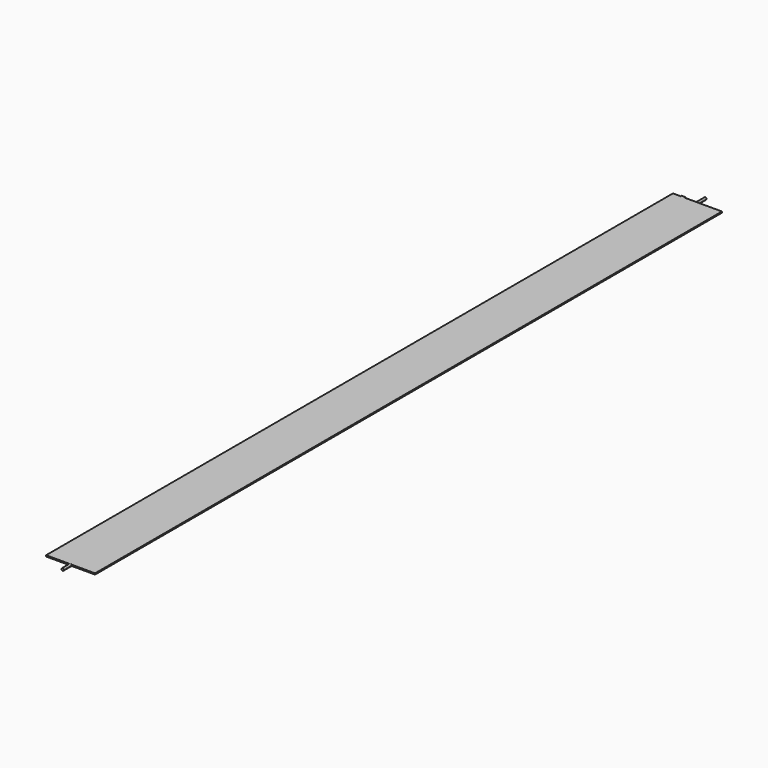
from build123d import *

# Parameters (mm, degrees)
F1_DEPTH = 3
F2_W     = 10
F2_H     = 3
F2_H_2   = 40
F2_R     = 1.5
F3_DEPTH = 3
F5_DEPTH = 25
F7_DEPTH = 25


# Not quite as in the source:
# - a feature names something its author has since deleted; it is built from what else it names


with BuildPart() as f1:
    # F0 (on Top) → F1 (new body)
    with BuildSketch(Plane.XY):
        Polygon((25.6095033884, 1855.804875493), (-34.3904966116, 1855.804875493), (-34.3904966116, -144.195124507), (25.6095033884, -144.195124507), (25.6095033884, -164.195124507), (30.6095033884, -164.195124507), (30.6095033884, -144.195124507), (90.6095033884, -144.195124507), (90.6095033884, 1855.804875493), (30.6095033884, 1855.804875493), (30.6095033884, 1875.804875493), (25.6095033884, 1875.804875493), align=None)
    extrude(amount=F1_DEPTH)

    # F2 (on face) → F3 (join)
    with BuildSketch(Plane(origin=(0, 1855.804875493, 0), x_dir=(-1, 0, 0), z_dir=(0, 1, 0))):
        with Locations((9.3904966116, 1.5)):
            Rectangle(F2_W, F2_H)
        with Locations((9.3904966116, -20)):
            Rectangle(F2_W, F2_H_2)
        with Locations((9.3904966116, -35)):
            Circle(F2_R, mode=Mode.SUBTRACT)
    extrude(amount=F3_DEPTH)

    # F4 (on face) → F5 (join)
    with BuildSketch(Plane.XZ.offset(144.195124507)):
        with BuildLine():
            Line((30.6095033884, 3), (30.7075795998, 3))
            ThreePointArc((30.7075795998, 3), (25.1095033884, 1.5), (30.7075795998, 0))
            Line((30.7075795998, 0), (30.6095033884, 0))
            Line((30.6095033884, 0), (30.6095033884, 3))
        make_face()
        with BuildLine():
            ThreePointArc((30.7075795998, 0), (31.0072808673, 0.7235428647), (31.1095033884, 1.5))
            ThreePointArc((31.1095033884, 1.5), (31.0072808673, 2.2764571353), (30.7075795998, 3))
            Line((30.7075795998, 3), (30.6095033884, 3))
            Line((30.6095033884, 3), (30.6095033884, 0))
            Line((30.6095033884, 0), (30.7075795998, 0))
        make_face()
    extrude(amount=F5_DEPTH)

    # F6 (on face) → F7 (join)
    with BuildSketch(Plane(origin=(0, 1855.804875493, 0), x_dir=(-1, 0, 0), z_dir=(0, 1, 0))):
        with BuildLine():
            Line((-30.6095033884, 3), (-30.7075795998, 3))
            ThreePointArc((-30.7075795998, 3), (-31.1095033884, 1.5), (-30.7075795998, 0))
            Line((-30.7075795998, 0), (-30.6095033884, 0))
            Line((-30.6095033884, 0), (-30.6095033884, 3))
        make_face()
        with BuildLine():
            ThreePointArc((-30.7075795998, 0), (-27.3330462531, -1.3977774789), (-25.1095033884, 1.5))
            ThreePointArc((-25.1095033884, 1.5), (-27.3330462531, 4.3977774789), (-30.7075795998, 3))
            Line((-30.7075795998, 3), (-30.6095033884, 3))
            Line((-30.6095033884, 3), (-30.6095033884, 0))
            Line((-30.6095033884, 0), (-30.7075795998, 0))
        make_face()
    extrude(amount=F7_DEPTH)


solid = f1.part
